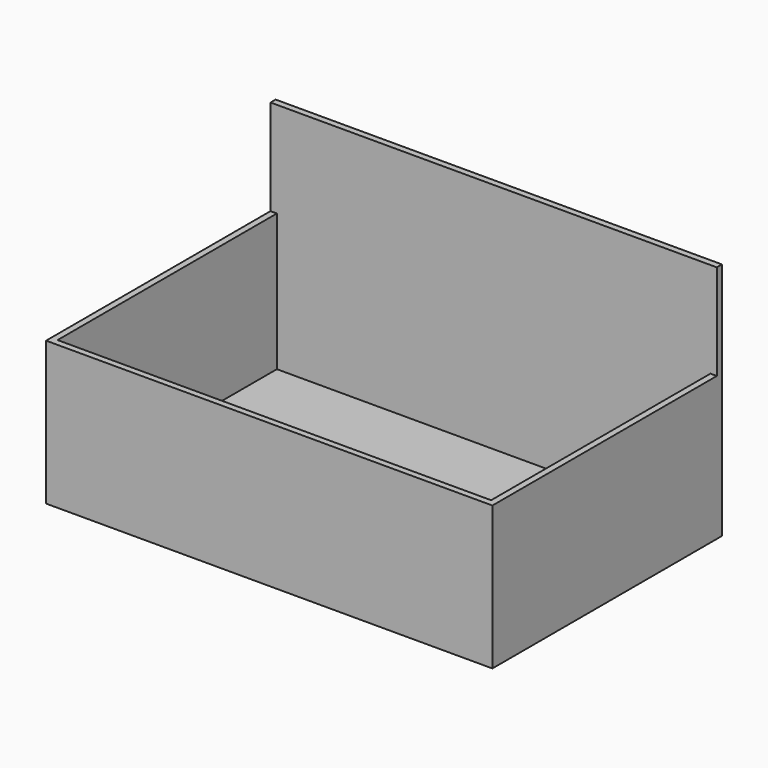
from build123d import *

# Parameters (mm, degrees)
F0_W     = 177.8
F0_H     = 114.3
F1_DEPTH = 57.15
F2_T     = -2.54
F4_DEPTH = 38.1


with BuildPart() as f1:
    # F0 (on Top) → F1 (new body)
    with BuildSketch(Plane.XY):
        with Locations((20.6855162978, 20.978878082)):
            Rectangle(F0_W, F0_H)
    extrude(amount=F1_DEPTH)

    # F2
    f2_openings = [f1.faces().sort_by_distance(p)[0] for p in [
        (20.685516, 20.978878, 57.15),
    ]]
    offset(amount=F2_T, openings=f2_openings)

    # F3 (on face) → F4 (join)
    with BuildSketch(Plane.XY.offset(57.15)):
        Polygon((-68.2144837022, 75.588878082), (-65.6744837022, 75.588878082), (107.0455162978, 75.588878082), (109.5855162978, 75.588878082), (109.5855162978, 78.128878082), (-68.2144837022, 78.128878082), align=None)
    extrude(amount=F4_DEPTH)


solid = f1.part
